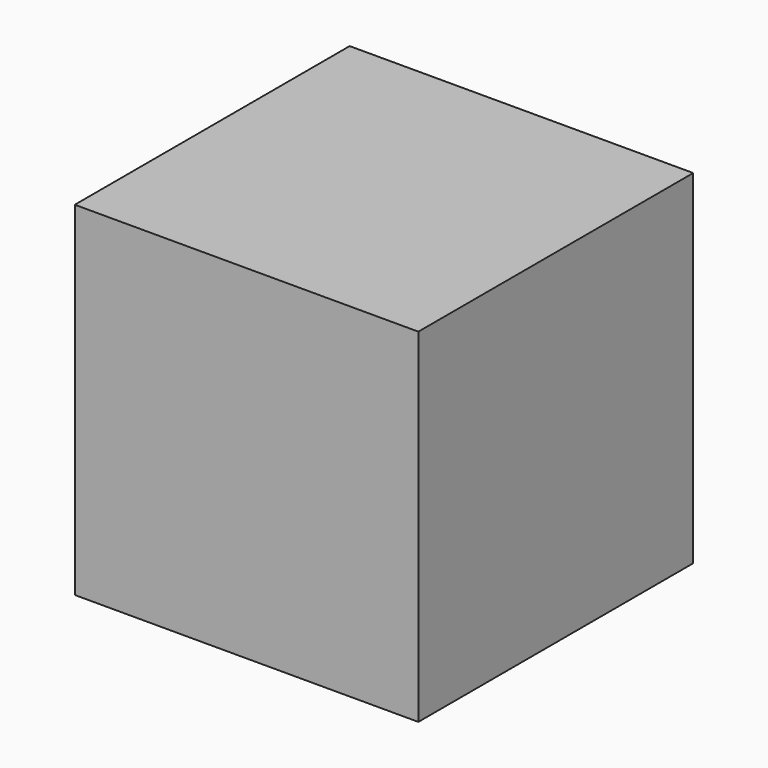
from build123d import *

# Parameters (mm, degrees)
F0_W     = 100
F0_H     = 100
F1_DEPTH = 100


# Not quite as in the source:
# - a feature of the source that left no trace in its solid (it failed there, or was rolled back) is left out


with BuildPart() as f1:
    # F0 (on Top) → F1 (new body)
    with BuildSketch(Plane.XY):
        Rectangle(F0_W, F0_H)
    extrude(amount=F1_DEPTH)


solid = f1.part
